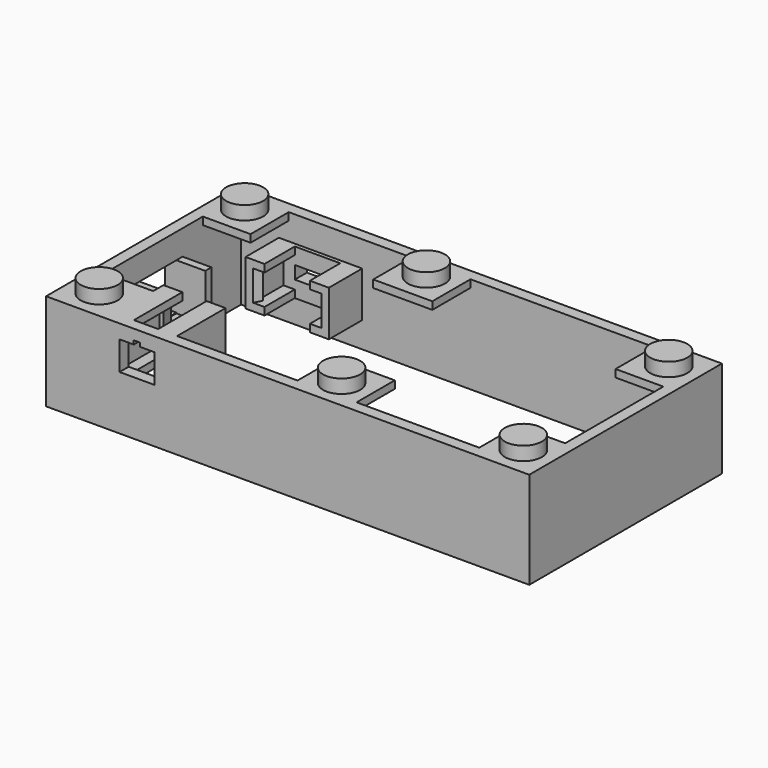
from build123d import *

# Parameters (mm, degrees)
F0_W      = 63.8
F0_H      = 31.8
F0_W_2    = 60.8
F0_H_2    = 28.8
F1_DEPTH  = 12.8
F2_W      = 6.3
F2_H      = 6.3
F2_W_2    = 7.8
F3_DEPTH  = 1
F4_R      = 2.45
F5_DEPTH  = 1.8
F6_W      = 0.85
F6_H      = 0.5
F7_DEPTH  = 25.4
F9_DEPTH  = 8
F11_DEPTH = 5
F12_W     = 0.1
F12_H     = 1
F13_DEPTH = 6.3
F14_W     = 6
F14_H     = 1.7
F15_DEPTH = 2.54
F16_W     = 11
F16_H     = 6
F16_W_2   = 6
F16_H_2   = 1.7
F17_DEPTH = 0.5
F19_DEPTH = 5
F21_DEPTH = 4
F22_W     = 6.096
F22_H     = 6.096
F23_DEPTH = 25.4
F24_W     = 1.0284033013
F24_H     = 6.0595651898
F25_DEPTH = 3.81
F26_W     = 1.0230291676
F26_H     = 6.1809321209
F27_DEPTH = 3.81
F28_W     = 8.1515833735
F28_H     = 1.3899055775
F29_DEPTH = 3.81


# Not quite as in the source:
# - a feature names something its author has since deleted; it is built from what else it names


with BuildPart() as f1:
    # F0 (on Top) → F1 (new body)
    with BuildSketch(Plane.XY):
        with Locations((31.9, 15.9)):
            Rectangle(F0_W, F0_H)
        with Locations((31.9, 15.9)):
            Rectangle(F0_W_2, F0_H_2, mode=Mode.SUBTRACT)
    extrude(amount=F1_DEPTH)

    # F2 (on face) → F3 (join)
    with BuildSketch(Plane.XY.offset(12.8)):
        with Locations((4.65, 27.15)):
            Rectangle(F2_W, F2_H)
        with Locations((4.65, 4.65)):
            Rectangle(F2_W, F2_H)
        with Locations((59.15, 4.65)):
            Rectangle(F2_W, F2_H)
        with Locations((59.15, 27.15)):
            Rectangle(F2_W, F2_H)
        with Locations((27.9, 27.15)):
            Rectangle(F2_W_2, F2_H)
        with Locations((35.9, 4.65)):
            Rectangle(F2_W_2, F2_H)
    extrude(amount=-F3_DEPTH)

    # F4 (on face) → F5 (join)
    with BuildSketch(Plane.XY.offset(12.8)):
        with Locations((3.9, 27.9)):
            Circle(F4_R)
        with Locations((59.9, 27.9)):
            Circle(F4_R)
        with Locations((59.9, 3.9)):
            Circle(F4_R)
        with Locations((3.9, 3.9)):
            Circle(F4_R)
        with Locations((27.9, 27.9)):
            Circle(F4_R)
        with Locations((35.9, 3.9)):
            Circle(F4_R)
    extrude(amount=F5_DEPTH)

    # F6 (on face) → F7 (cut)
    with BuildSketch(Plane.XZ):
        Polygon((11.575, 10.95), (9.7, 10.95), (9.7, 7.15), (14.3, 7.15), (14.3, 10.95), (12.425, 10.95), align=None)
        with Locations((12, 11.2)):
            Rectangle(F6_W, F6_H)
    extrude(amount=-F7_DEPTH, mode=Mode.SUBTRACT)

    # F8 (on face) → F9 (join)
    with BuildSketch(Plane(origin=(0, 1.5, 0), x_dir=(-1, 0, 0), z_dir=(0, 1, 0))):
        Polygon((-13.6, 5.8), (-13.6, 6.8), (-15.1, 6.8), (-15.1, 11.8), (-13.6, 11.8), (-13.6, 12.8), (-16.1, 12.8), (-16.1, 5.8), align=None)
        Polygon((-8.9, 6.8), (-10.4, 6.8), (-10.4, 5.8), (-7.9, 5.8), (-7.9, 12.8), (-10.4, 12.8), (-10.4, 11.8), (-8.9, 11.8), align=None)
    extrude(amount=F9_DEPTH)

    # F10 (on face) → F11 (join, through all)
    with BuildSketch(Plane.XY.offset(6.8)):
        Polygon((14.6, 7.6), (15.1, 7.6), (15.1, 9.5), align=None)
        Polygon((9.4, 7.6), (8.9, 9.5), (8.9, 7.6), align=None)
    extrude(amount=F11_DEPTH)

    # F12 (on face) → F13 (join, through all)
    with BuildSketch(Plane(origin=(0, 1.5, 0), x_dir=(-1, 0, 0), z_dir=(0, 1, 0))):
        with Locations((-7.85, 12.3)):
            Rectangle(F12_W, F12_H)
    extrude(amount=F13_DEPTH)

    # F14 (on face) → F15 (cut)
    with BuildSketch(Plane(origin=(0, 31.8, 0), x_dir=(-1, 0, 0), z_dir=(0, 1, 0))):
        with Locations((-12, 6.4)):
            Rectangle(F14_W, F14_H)
    extrude(amount=-F15_DEPTH, mode=Mode.SUBTRACT)

    # F16 (on face) → F17 (join)
    with BuildSketch(Plane.XZ.offset(-30.3)):
        with Locations((12, 6.4)):
            Rectangle(F16_W, F16_H)
        with Locations((12, 6.4)):
            Rectangle(F16_W_2, F16_H_2, mode=Mode.SUBTRACT)
    extrude(amount=F17_DEPTH)

    # F18 (on face) → F19 (join)
    with BuildSketch(Plane.XZ.offset(-29.8)):
        Polygon((9, 9.4), (6.5, 9.4), (6.5, 3.4), (9, 3.4), (9, 4.4), (7.5, 4.4), (7.5, 8.4), (9, 8.4), align=None)
        Polygon((17.5, 9.4), (15, 9.4), (15, 8.4), (16.5, 8.4), (16.5, 4.4), (15, 4.4), (15, 3.4), (17.5, 3.4), align=None)
    extrude(amount=F19_DEPTH)

    # F20 (on face) → F21 (join, through all)
    with BuildSketch(Plane.XY.offset(4.4)):
        Polygon((7.5, 25.8), (7.5, 24.8), (8, 25.8), align=None)
        Polygon((16, 25.8), (16.5, 24.8), (16.5, 25.8), align=None)
    extrude(amount=F21_DEPTH)

    # F22 (on face) → F23 (cut)
    with BuildSketch(Plane(origin=(0, 0, 0), x_dir=(0, -1, 0), z_dir=(-1, 0, 0))):
        with Locations((-16.5878270902, 6.4446975011)):
            Rectangle(F22_W, F22_H)
    extrude(amount=-F23_DEPTH, mode=Mode.SUBTRACT)

    # F24 (on face) → F25 (join)
    with BuildSketch(Plane.YZ.offset(1.5)):
        with Locations((13.0256254396, 6.4629149062)):
            Rectangle(F24_W, F24_H)
    extrude(amount=F25_DEPTH)

    # F26 (on face) → F27 (join)
    with BuildSketch(Plane.YZ.offset(1.5)):
        with Locations((20.147341674, 6.4022314407)):
            Rectangle(F26_W, F26_H)
    extrude(amount=F27_DEPTH)

    # F28 (on face) → F29 (join)
    with BuildSketch(Plane.YZ.offset(1.5)):
        with Locations((16.583064571, 2.6168125914)):
            Rectangle(F28_W, F28_H)
    extrude(amount=F29_DEPTH)


solid = f1.part
